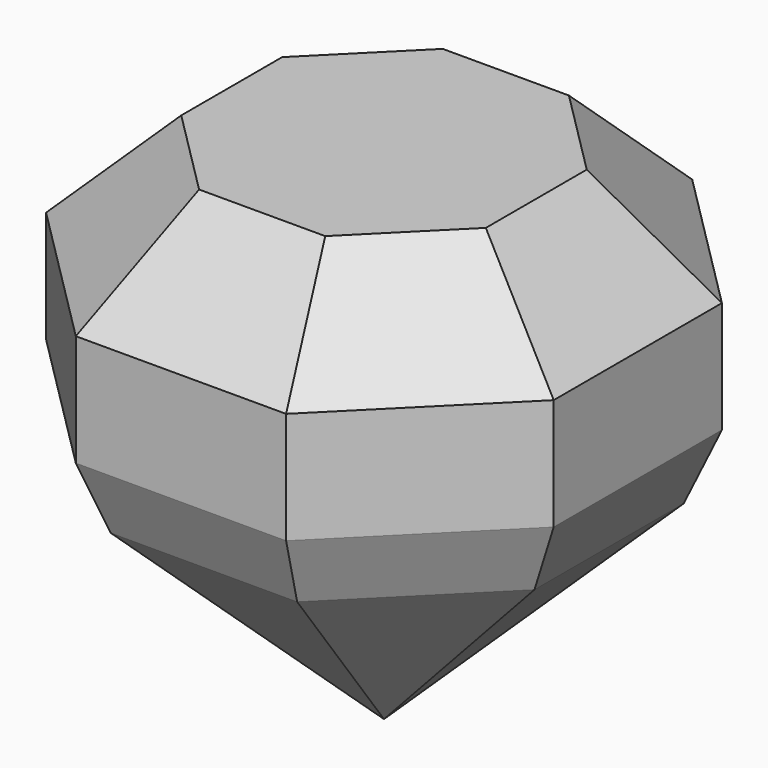
from build123d import *

# Parameters (mm, degrees)
F1_DEPTH = 25.4
F2_SIZE  = 12.7
F3_DEPTH = 38.1
F4_SIZE  = 31.7499
F5_SIZE  = 5.08


# Not quite as in the source:
# - a fillet or chamfer is up to 0.001 mm smaller than in the source, because OpenCascade refuses the exact size


with BuildPart() as f1:
    # F0 (on Top) → F1 (new body)
    with BuildSketch(Plane.XY):
        Polygon((31.75, -13.1512806053), (31.75, 13.1512806053), (13.1512806053, 31.75), (-13.1512806053, 31.75), (-31.75, 13.1512806053), (-31.75, -13.1512806053), (-13.1512806053, -31.75), (13.1512806053, -31.75), align=None)
    extrude(amount=F1_DEPTH)

    # F2
    f2_edges = [f1.edges().sort_by_distance(p)[0] for p in [
        (-31.75, 0, 25.4),
        (-22.45064, -22.45064, 25.4),
        (0, -31.75, 25.4),
        (22.45064, -22.45064, 25.4),
        (31.75, 0, 25.4),
        (22.45064, 22.45064, 25.4),
        (0, 31.75, 25.4),
        (-22.45064, 22.45064, 25.4),
    ]]
    chamfer(f2_edges, length=F2_SIZE)

    # F3 (add): a face of the model
    f3_faces = [f1.faces().sort_by_distance(p)[0] for p in [
        (0, 0, 0),
    ]]
    extrude(f3_faces, amount=F3_DEPTH)

    # F4 (size 31.75 in the source; OpenCascade refuses exactly that, so slightly less here)
    f4_edges = [f1.edges().sort_by_distance(p)[0] for p in [
        (-22.45064, -22.45064, -38.1),
        (0, -31.75, -38.1),
        (22.45064, -22.45064, -38.1),
        (-31.75, 0, -38.1),
        (-22.45064, 22.45064, -38.1),
        (0, 31.75, -38.1),
        (22.45064, 22.45064, -38.1),
        (31.75, 0, -38.1),
    ]]
    chamfer(f4_edges, length=F4_SIZE)

    # F5
    f5_edges = [f1.edges().sort_by_distance(p)[0] for p in [
        (-31.75, 0, -6.3501),
        (-22.45064, 22.45064, -6.3501),
        (-22.45064, -22.45064, -6.3501),
        (0, -31.75, -6.3501),
        (22.45064, -22.45064, -6.3501),
        (31.75, 0, -6.3501),
        (22.45064, 22.45064, -6.3501),
        (0, 31.75, -6.3501),
    ]]
    chamfer(f5_edges, length=F5_SIZE)


solid = f1.part
